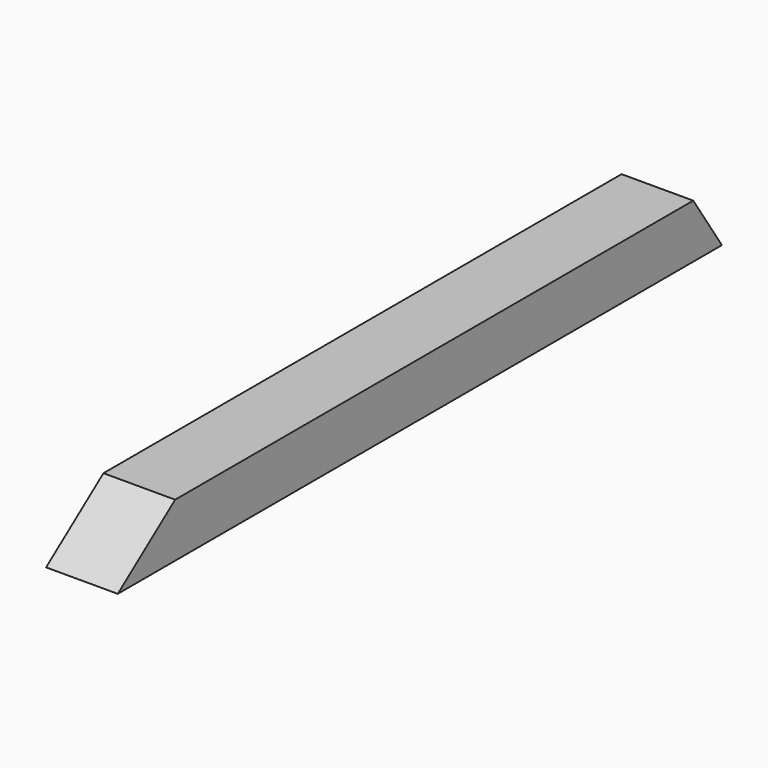
from build123d import *

# Parameters (mm, degrees)
F0_W     = 30
F0_H     = 316
F1_DEPTH = 5
F2_DEPTH = 17.5
F3_SIZE2 = 14.99999
F3_SIZE  = 22.49999
F4_SIZE2 = 22.49999
F4_SIZE  = 29.99999
F5_T     = 2.5
F6_DEPTH = 25
F7_DEPTH = 2.4


# Not quite as in the source:
# - a fillet or chamfer is up to 0.001 mm smaller than in the source, because OpenCascade refuses the exact size
# - a shell that OpenCascade refuses in one call is made with other operations: the cavity is built on its own and cut out


with BuildPart() as f1:
    # F0 (on Top) → F1 (new body)
    with BuildSketch(Plane.XY):
        Rectangle(F0_W, F0_H)
    extrude(amount=F1_DEPTH)

    # F2 (add): a face of the model
    f2_faces = [f1.faces().sort_by_distance(p)[0] for p in [
        (0, 0, 0),
    ]]
    extrude(f2_faces, amount=F2_DEPTH)

    # F3 (size 22.5 and 15 in the source; OpenCascade refuses exactly that, so slightly less here)
    f3_edges = [f1.edges().sort_by_distance(p)[0] for p in [
        (0, 158, 5),
    ]]
    f3_side = f1.faces().sort_by_distance((0, 158, -6.25))[0]
    chamfer(f3_edges, length=F3_SIZE, length2=F3_SIZE2, reference=f3_side)

    # F4 (size 30 and 22.5 in the source; OpenCascade refuses exactly that, so slightly less here)
    f4_edges = [f1.edges().sort_by_distance(p)[0] for p in [
        (0, -158, 5),
    ]]
    f4_side = f1.faces().sort_by_distance((0, -7.499995, 5))[0]
    chamfer(f4_edges, length=F4_SIZE, length2=F4_SIZE2, reference=f4_side)

    # F5: shell of thickness 2.5, made by hand


with BuildPart() as f5_core1:
    # F5_t2: copy of F1
    add(f1.part)

    # the walls: a layer under each face that stays
    f5_faces = [f5_core1.faces().sort_by_distance(p)[0] for p in [
        (15, 0, -6.25),
        (0, 7.5, 5),
        (0, -143.000005, -6.249995),
        (0, 150.500005, -6.249995),
        (0, -158, -17.499995),
        (0, 158, -17.499995),
        (-15, 0, -6.25),
    ]]
    thicken(f5_faces, amount=-F5_T, mode=Mode.SUBTRACT)


with BuildPart() as f1_1:
    add(f1.part)

    # what is left inside the walls is the cavity
    f5_cavity = [f5_core1.part.solids().sort_by_distance(p)[0] for p in [
        (0, -50.890437, -17.475),
    ]]
    add(f5_cavity, mode=Mode.SUBTRACT)

    # F6 (cut): a face of the model
    f6_faces = [f1_1.faces().sort_by_distance(p)[0] for p in [
        (-12.5, 3.8374129004, -7.7308172989),
    ]]
    extrude(f6_faces, amount=-F6_DEPTH, mode=Mode.SUBTRACT)

    # F7 (cut): a face of the model
    f7_faces = [f1_1.faces().sort_by_distance(p)[0] for p in [
        (12.5, 3.8374129004, -7.7308172989),
    ]]
    extrude(f7_faces, amount=-F7_DEPTH, mode=Mode.SUBTRACT)


solid = f1_1.part
